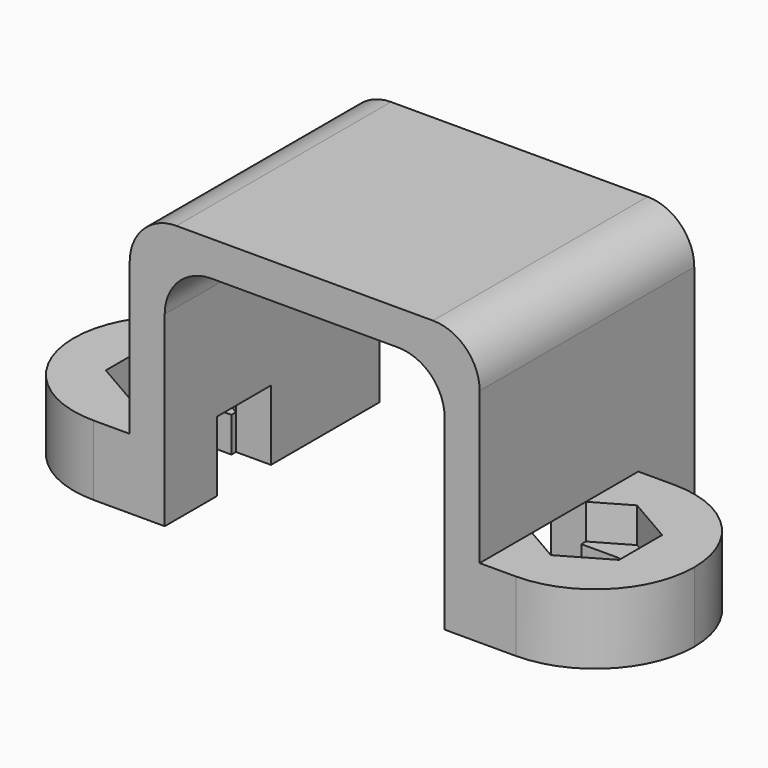
from build123d import *

# Parameters (mm, degrees)
F0_W     = 1.5
F0_H     = 2.806624327
F1_DEPTH = 11.5
F2_DEPTH = 10
F3_DEPTH = 3
F4_DEPTH = 3
F5_DEPTH = 1.5
F6_R     = 4.24999
F7_R     = 2


# Not quite as in the source:
# - a fillet or chamfer is up to 0.001 mm smaller than in the source, because OpenCascade refuses the exact size


with BuildPart() as f1:
    # F0 (on Top) → F1 (new body)
    with BuildSketch(Plane.XY):
        Polygon((-6, 7.25), (-6, 1.443375673), (-6, -1.443375673), (-6, -4.25), (0, -4.25), (0, 7.25), align=None)
        Polygon((-7.5, 4.25), (-7.5, 1.443375673), (-6, 1.443375673), (-6, 7.25), (-7.5, 7.25), align=None)
        Polygon((-7.5, 1.443375673), (-7.5, 1.1999995727), (-7.5, -1.1999995727), (-7.5, -1.443375673), (-6, -1.443375673), (-6, 1.443375673), align=None)
        with Locations((-6.75, -2.8466878365)):
            Rectangle(F0_W, F0_H)
        Polygon((6, 7.25), (0, 7.25), (0, -4.25), (6, -4.25), (6, -1.443375673), (6, 1.443375673), align=None)
        Polygon((7.5, 7.25), (6, 7.25), (6, 1.443375673), (7.5, 1.443375673), (7.5, 4.25), align=None)
        Polygon((7.5, 1.443375673), (6, 1.443375673), (6, -1.443375673), (7.5, -1.443375673), (7.5, -1.1999995727), (7.5, 1.1999995727), align=None)
        with Locations((6.75, -2.8466878365)):
            Rectangle(F0_W, F0_H)
    extrude(amount=F1_DEPTH)

    # F0 (on Top) → F2 (cut)
    with BuildSketch(Plane.XY):
        Polygon((-6, 7.25), (-6, 1.443375673), (-6, -1.443375673), (-6, -4.25), (0, -4.25), (0, 7.25), align=None)
        Polygon((6, 7.25), (0, 7.25), (0, -4.25), (6, -4.25), (6, -1.443375673), (6, 1.443375673), align=None)
    extrude(amount=F2_DEPTH, mode=Mode.SUBTRACT)

    # F0 (on Top) → F3 (cut)
    with BuildSketch(Plane.XY):
        Polygon((-7.5, 1.443375673), (-7.5, 1.1999995727), (-7.5, -1.1999995727), (-7.5, -1.443375673), (-6, -1.443375673), (-6, 1.443375673), align=None)
        Polygon((7.5, 1.443375673), (6, 1.443375673), (6, -1.443375673), (7.5, -1.443375673), (7.5, -1.1999995727), (7.5, 1.1999995727), align=None)
    extrude(amount=F3_DEPTH, mode=Mode.SUBTRACT)

    # F0 (on Top) → F4 (join)
    with BuildSketch(Plane.XY):
        Polygon((-9, 2.3094010768), (-7.5, 1.443375673), (-7.5, 4.25), (-13.3, 4.25), (-13.3, -4.25), (-7.5, -4.25), (-7.5, -1.443375673), (-9, -2.3094010768), (-11, -1.1547005384), (-11, 1.1547005384), align=None)
        Polygon((7.5, -1.443375673), (7.5, -4.25), (13.3, -4.25), (13.3, 4.25), (7.5, 4.25), (7.5, 1.443375673), (9, 2.3094010768), (11, 1.1547005384), (11, -1.1547005384), (9, -2.3094010768), align=None)
    extrude(amount=F4_DEPTH)

    # F0 (on Top) → F5 (join)
    with BuildSketch(Plane.XY):
        with BuildLine():
            ThreePointArc((-9, -1.1999995727), (-10.1999995727, 0), (-9, 1.1999995727))
            Line((-9, 1.1999995727), (-7.5, 1.1999995727))
            Line((-7.5, 1.1999995727), (-7.5, 1.443375673))
            Line((-7.5, 1.443375673), (-9, 2.3094010768))
            Line((-9, 2.3094010768), (-11, 1.1547005384))
            Line((-11, 1.1547005384), (-11, -1.1547005384))
            Line((-11, -1.1547005384), (-9, -2.3094010768))
            Line((-9, -2.3094010768), (-7.5, -1.443375673))
            Line((-7.5, -1.443375673), (-7.5, -1.1999995727))
            Line((-7.5, -1.1999995727), (-9, -1.1999995727))
        make_face()
        with BuildLine():
            Line((9, 2.3094010768), (7.5, 1.443375673))
            Line((7.5, 1.443375673), (7.5, 1.1999995727))
            Line((7.5, 1.1999995727), (9, 1.1999995727))
            ThreePointArc((9, 1.1999995727), (10.1999995727, 0), (9, -1.1999995727))
            Line((9, -1.1999995727), (7.5, -1.1999995727))
            Line((7.5, -1.1999995727), (7.5, -1.443375673))
            Line((7.5, -1.443375673), (9, -2.3094010768))
            Line((9, -2.3094010768), (11, -1.1547005384))
            Line((11, -1.1547005384), (11, 1.1547005384))
            Line((11, 1.1547005384), (9, 2.3094010768))
        make_face()
    extrude(amount=F5_DEPTH)

    # F6 (radius 4.25 in the source; OpenCascade refuses exactly that, so slightly less here)
    f6_edges = [f1.edges().sort_by_distance(p)[0] for p in [
        (-13.3, -4.25, 1.5),
        (-13.3, 4.25, 1.5),
        (13.3, 4.25, 1.5),
        (13.3, -4.25, 1.5),
    ]]
    fillet(f6_edges, radius=F6_R)

    # F7
    f7_edges = [f1.edges().sort_by_distance(p)[0] for p in [
        (6, 1.5, 10),
        (7.5, 1.5, 11.5),
        (-7.5, 1.5, 11.5),
        (-6, 1.5, 10),
    ]]
    fillet(f7_edges, radius=F7_R)


solid = f1.part
